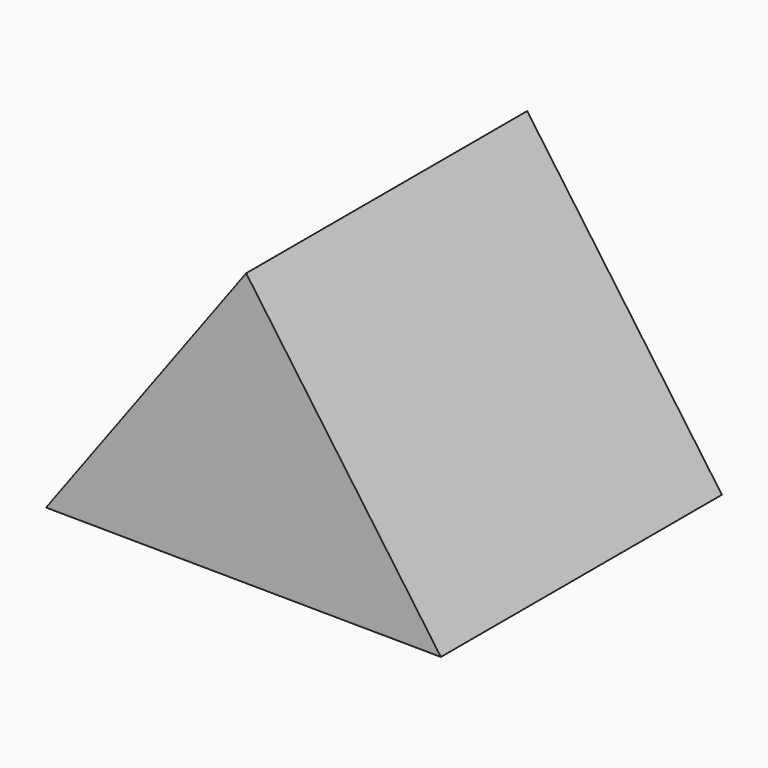
from build123d import *

# Parameters (mm, degrees)
F1_DEPTH     = 100
F2_TEXT_SIZE = 6.679388591
F3_DEPTH     = 25


# Not quite as in the source:
# - Text() gives the source's letters only with a copy of the font that has no kerning and outlines rounded to 1/6400 em; it was checked with that copy


with BuildPart() as f1:
    # F0 (on Front) → F1 (new body)
    with BuildSketch(Plane.XZ):
        Polygon((55.4343946278, -24.7921794653), (0, 53.3516258001), (-56.9584928453, -23.8955169916), align=None)
    extrude(amount=F1_DEPTH)

    # F2 (on face) → F3 (cut)
    with BuildSketch(Plane(origin=(0, 0, 0), x_dir=(-1, 0, 0), z_dir=(0, 1, 0))):
        with Locations((-6.4623090439, 21.1903639138)):
            Text('JV', F2_TEXT_SIZE, font='Open Sans', text_align=(TextAlign.LEFT, TextAlign.BOTTOM))
    extrude(amount=-F3_DEPTH, mode=Mode.SUBTRACT)


solid = f1.part
